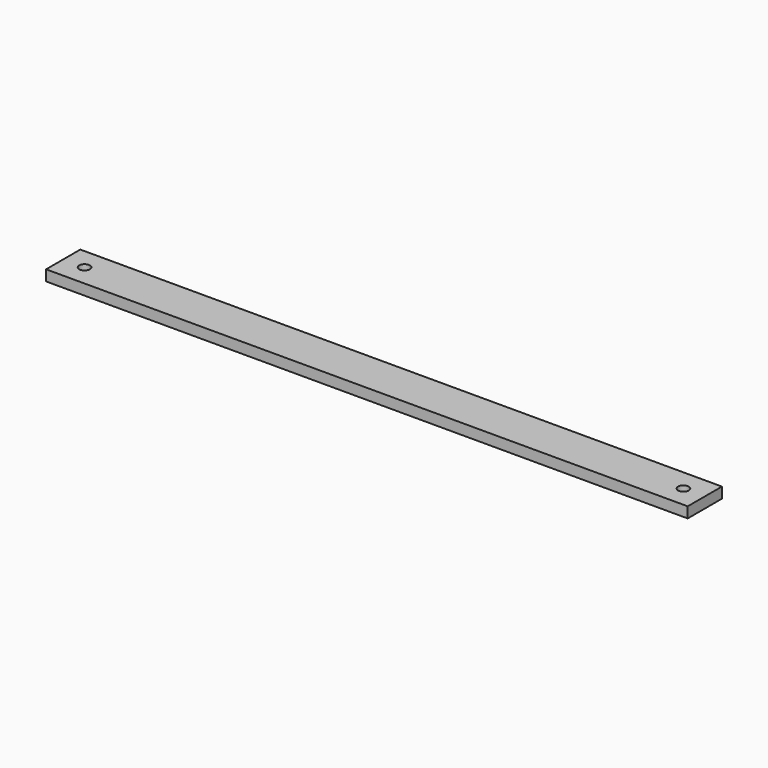
from build123d import *

# Parameters (mm, degrees)
F0_W     = 381
F0_H     = 25.4
F1_DEPTH = 6.35
F2_R     = 3.175
F3_DEPTH = 25.4


# Not quite as in the source:
# - a feature names something its author has since deleted; it is built from what else it names


with BuildPart() as f1:
    # F0 (on Top) → F1 (new body)
    with BuildSketch(Plane.XY):
        Rectangle(F0_W, F0_H)
    extrude(amount=F1_DEPTH)

    # F2 (on face) → F3 (cut)
    with BuildSketch(Plane.XY.offset(6.35)):
        with Locations((-177.8, 0)):
            Circle(F2_R)
        with Locations((177.8, 0)):
            Circle(F2_R)
    extrude(amount=-F3_DEPTH, mode=Mode.SUBTRACT)


solid = f1.part
